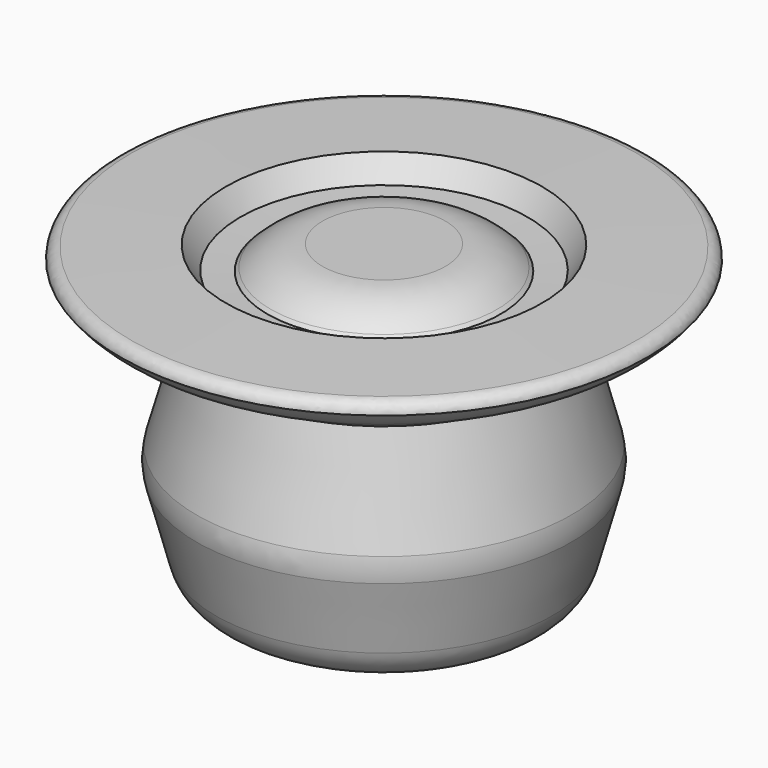
from build123d import *

# Parameters (mm, degrees)
F2_R = 5
F3_R = 0.7471384798
F5_R = 3.0872818621


# Not quite as in the source:
# - a fillet or chamfer that OpenCascade refuses, or shapes differently, is made with other operations: its cross-section is extruded or revolved along the edge and cut away or added


with BuildPart() as f1:
    # F0 (on Front) → F1 (revolve)
    with BuildSketch(Plane.XZ):
        Polygon((-10.6199271977, 0), (0, 0), (0, 20.5089394003), (-6.1166980304, 20.5089394003), (-7.7893259004, 18.9006421715), (-9.590617381, 18.9649742097), (-10.5555951595, 20.4446054995), (-17.6320988685, 20.3159432858), (-17.6320988685, 19.0936364233), (-10.748591274, 15.3623912483), (-12.7428779379, 7.8355651349), align=None)
    revolve(axis=Axis((0, 0, 10.2544697002), (0, 0, -1)))

    # F2
    f2_edges = [f1.edges().sort_by_distance(p)[0] for p in [
        (6.116698, 0, 20.508939),
    ]]
    fillet(f2_edges, radius=F2_R)

    # F3
    f3_edges = [f1.edges().sort_by_distance(p)[0] for p in [
        (17.632099, 0, 20.315943),
    ]]
    fillet(f3_edges, radius=F3_R)

    # F4: fillet of radius 5 on 1 edges, made by hand

    # F4_s1 → F4_t2 (revolve, cut)
    with BuildSketch(Plane.XZ):
        with BuildLine():
            ThreePointArc((-17.6320943676, 19.5822655038), (-16.9135613616, 18.827647757), (-16.0542267415, 18.2383416946))
            Line((-16.0542267415, 18.2383416946), (-17.6320988685, 19.0936364233))
            ThreePointArc((-17.6320988685, 19.0936364233), (-17.6320988685, 19.3379509636), (-17.6320943676, 19.5822655038))
        make_face()
    revolve(axis=Axis((0, 0, 19.0936364233), (0, 0, -1)), mode=Mode.SUBTRACT)

    # F5
    f5_edges = [f1.edges().sort_by_distance(p)[0] for p in [
        (12.742878, 0, 7.835565),
        (10.619927, 0, 0),
        (-11.681403, 0, 3.917783),
    ]]
    fillet(f5_edges, radius=F5_R)


solid = f1.part
